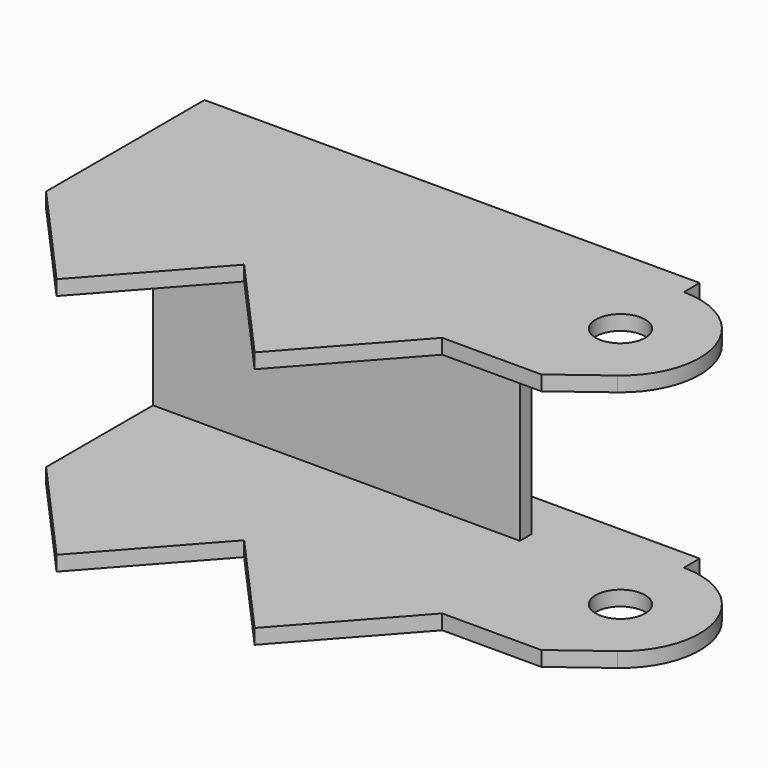
from build123d import *

# Parameters (mm, degrees)
F0_R     = 5
F1_DEPTH = 52
F2_W     = 31.6232873572
F2_H     = 46
F2_W_2   = 27
F2_W_3   = 8.3583824264
F2_W_4   = 10
F3_DEPTH = 116.001
F4_R     = 2.99999
F5_W     = 50
F5_H     = 46
F6_DEPTH = 52.361679775


# Not quite as in the source:
# - a fillet or chamfer is up to 0.001 mm smaller than in the source, because OpenCascade refuses the exact size


with BuildPart() as f1:
    # F0 (on Top) → F1 (new body)
    with BuildSketch(Plane.XY):
        with BuildLine():
            Line((15.0605264698, 33.6507520748), (15.0605264698, 37.6507520748))
            Line((15.0605264698, 37.6507520748), (-84.9394735302, 37.6507520748))
            Line((-84.9394735302, 37.6507520748), (-84.9394735302, -2.3492479252))
            Line((-84.9394735302, -2.3492479252), (-64.9394735302, -24.7099277002))
            Line((-64.9394735302, -24.7099277002), (-44.9394735302, -2.3492479252))
            Line((-44.9394735302, -2.3492479252), (-24.9394735302, -24.7099277002))
            Line((-24.9394735302, -24.7099277002), (-4.9394735302, -2.3492479252))
            Line((-4.9394735302, -2.3492479252), (15.0605264698, -2.3492479252))
            Line((15.0605264698, -2.3492479252), (24.6605264698, 4.8507520748))
            ThreePointArc((24.6605264698, 4.8507520748), (30.2394592386, 22.7103963311), (15.0605264698, 33.6507520748))
        make_face()
        with Locations((15.0605264698, 17.6507520748)):
            Circle(F0_R, mode=Mode.SUBTRACT)
    extrude(amount=F1_DEPTH)

    # F2 (on face) → F3 (cut, through all)
    with BuildSketch(Plane(origin=(-84.9394735302, 0, 0), x_dir=(0, -1, 0), z_dir=(-1, 0, 0))):
        with Locations((18.1608916038, 26)):
            Rectangle(F2_W, F2_H)
        with Locations((-11.1507520748, 26)):
            Rectangle(F2_W_2, F2_H)
        with Locations((-41.829943288, 26)):
            Rectangle(F2_W_3, F2_H)
        with Locations((-32.6507520748, 26)):
            Rectangle(F2_W_4, F2_H)
    extrude(amount=-F3_DEPTH, mode=Mode.SUBTRACT)

    # F4 (radius 3 in the source; OpenCascade refuses exactly that, so slightly less here)
    f4_edges = [f1.edges().sort_by_distance(p)[0] for p in [
        (27.550522, 27.650752, 26),
        (-84.939474, 27.650752, 26),
    ]]
    fillet(f4_edges, radius=F4_R)

    # F5 (on face) → F6 (cut, through all)
    with BuildSketch(Plane(origin=(0, 27.6507520748, 0), x_dir=(-1, 0, 0), z_dir=(0, 1, 0))):
        with Locations((-14.1408709809, 26)):
            Rectangle(F5_W, F5_H)
    extrude(amount=-F6_DEPTH, mode=Mode.SUBTRACT)


solid = f1.part
